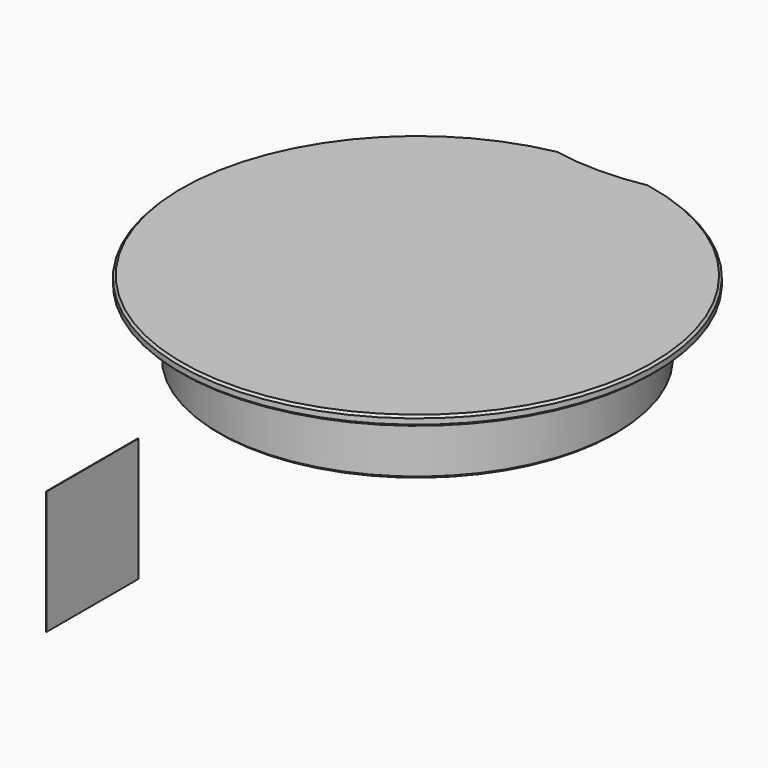
from build123d import *

# Parameters (mm, degrees)
F0_R     = 36.5
F0_R_2   = 34.9
F1_DEPTH = 1.8
F2_DEPTH = 12
F3_R     = 34.9
F3_R_2   = 31.9
F4_DEPTH = 7
F5_SIZE  = 2.99999
F6_W     = 21.030202508
F6_H     = 22.6074543316
F7_DEPTH = 0.1
F8_SIZE  = 0.4


# Not quite as in the source:
# - a fillet or chamfer is up to 0.001 mm smaller than in the source, because OpenCascade refuses the exact size


with BuildPart() as f1:
    # F0 (on Top) → F1 (new body)
    with BuildSketch(Plane.XY):
        with BuildLine():
            ThreePointArc((-9.2736184955, 42.5), (-27.2841308772, -33.8795838563), (43.5, 0))
            ThreePointArc((43.5, 0), (33.8795838563, 27.2841308772), (9.2736184955, 42.5))
            ThreePointArc((9.2736184955, 42.5), (0, 41.5), (-9.2736184955, 42.5))
        make_face()
        Circle(F0_R, mode=Mode.SUBTRACT)
        Circle(F0_R)
        Circle(F0_R_2, mode=Mode.SUBTRACT)
        Circle(F0_R_2)
    extrude(amount=F1_DEPTH)

    # F0 (on Top) → F2 (join)
    with BuildSketch(Plane.XY):
        Circle(F0_R)
        Circle(F0_R_2, mode=Mode.SUBTRACT)
    extrude(amount=-F2_DEPTH)

    # F3 (on face) → F4 (join)
    with BuildSketch(Plane(origin=(0, 0, -12), x_dir=(1, 0, 0), z_dir=(0, 0, -1))):
        Circle(F3_R)
        Circle(F3_R_2, mode=Mode.SUBTRACT)
    extrude(amount=-F4_DEPTH)

    # F5 (size 3 in the source; OpenCascade refuses exactly that, so slightly less here)
    f5_edges = [f1.edges().sort_by_distance(p)[0] for p in [
        (-31.9, 0, -12),
        (-31.9, 0, -5),
    ]]
    chamfer(f5_edges, length=F5_SIZE)

    # F8
    f8_edges = [f1.edges().sort_by_distance(p)[0] for p in [
        (0, -43.5, 1.8),
        (-36.5, 0, -12),
        (0, -43.5, 0),
    ]]
    chamfer(f8_edges, length=F8_SIZE)


with BuildPart() as f7:
    # F6 (on Right) → F7 (new body)
    with BuildSketch(Plane.YZ):
        with Locations((-74.3868201971, -9.776847437)):
            Rectangle(F6_W, F6_H)
    extrude(amount=F7_DEPTH)


solid = Compound([f1.part, f7.part])
